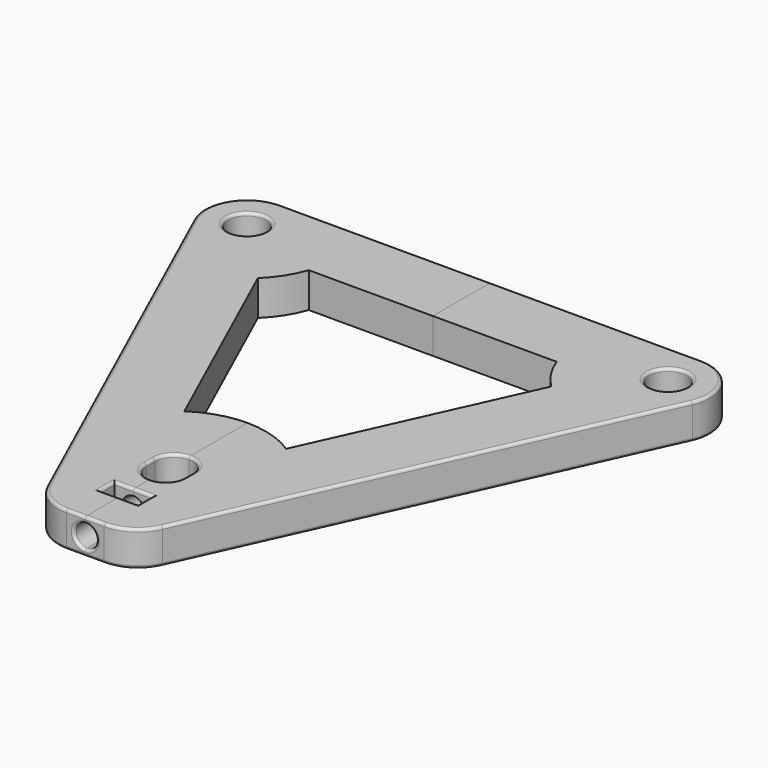
from build123d import *
from build123d import SkipClean  # not in build123d's __all__

# Parameters (mm, degrees)
F0_R          = 2.7
F1_DEPTH      = 5
F3_DEPTH      = 5
F5_END_RADIUS = 2.7
F4_R          = 1.6
F5_REACH      = 76.8264833996
F6_R          = 0.4


with BuildPart() as f1:
    # F0 (on Top) → F1 (new body)
    with BuildSketch(Plane.XY):
        with BuildLine():
            Line((0, -26.9), (0, 26.9))
            Line((0, 26.9), (-30, 26.9))
            ThreePointArc((-30, 26.9), (-35.0422077109, 24.1520979998), (-35.4659178703, 18.4253804667))
            Line((-35.4659178703, 18.4253804667), (-8.1659178703, -41.8746195333))
            ThreePointArc((-8.1659178703, -41.8746195333), (-5.9520979998, -44.4422077109), (-2.7, -45.4))
            Line((-2.7, -45.4), (0, -45.4))
            Line((0, -45.4), (0, -39.4))
            Line((0, -39.4), (-2.7, -39.4))
            Line((-2.7, -39.4), (-2.7, -36.8))
            Line((-2.7, -36.8), (0, -36.8))
            Line((0, -36.8), (0, -33.8))
            ThreePointArc((0, -33.8), (-1.9091883092, -33.0091883092), (-2.7, -31.1))
            Line((-2.7, -31.1), (-2.7, -29.6))
            ThreePointArc((-2.7, -29.6), (-1.9091883092, -27.6908116908), (0, -26.9))
        make_face()
        with Locations((-30, 20.9)):
            Circle(F0_R, mode=Mode.SUBTRACT)
    extrude(amount=F1_DEPTH)

    # F2 (on face) → F3 (cut, through all)
    with BuildSketch(Plane.XY.offset(5)):
        with BuildLine():
            Line((0, -16.5), (0, 16.5))
            Line((0, 16.5), (-17.6610373207, 16.5))
            ThreePointArc((-17.6610373207, 16.5), (-18.9911798312, 13.7995860339), (-20.9026205506, 11.4740948895))
            Line((-20.9026205506, 11.4740948895), (-7.2474182596, -18.687395885))
            ThreePointArc((-7.2474182596, -18.687395885), (-3.7851609011, -17.0587657325), (0, -16.5))
        make_face()
    extrude(amount=-F3_DEPTH, mode=Mode.SUBTRACT)

    f5_end = (Plane(origin=(0, -31.1, 2.5), x_dir=(-1, 0, 0), z_dir=(0, 0, -1)) * Cylinder(F5_END_RADIUS, 315.4959771518, mode=Mode.PRIVATE)).faces().sort_by_distance((-1.9091883092, -33.0091883092, 2.5))[0]
    # F4 (on face) → F5 (cut, up to the whole of a round face its end follows)
    with BuildSketch(Plane.XZ.offset(45.4)):
        with Locations((0, 2.5)):
            Circle(F4_R)
    f5_long = extrude(amount=-F5_REACH, mode=Mode.PRIVATE)
    add(split(f5_long, bisect_by=f5_end, keep=Keep.ALL, mode=Mode.PRIVATE).solids().sort_by_distance((0, -45.4, 2.5))[0], mode=Mode.SUBTRACT)

    # F6
    f6_edges = [f1.edges().sort_by_distance(p)[0] for p in [
        (-21.815918, -11.72462, 5),
        (-5.952098, -44.442208, 0),
        (-1.6, -45.4, 2.5),
        (-2.7, -38.1, 5),
        (-1.35, -39.4, 5),
        (-1.35, -36.8, 5),
        (-1.35, -39.4, 0),
        (-2.7, -38.1, 0),
        (-1.35, -36.8, 0),
        (-32.7, 20.9, 5),
        (-32.7, 20.9, 0),
        (-1.909188, -33.009188, 0),
        (-2.7, -30.35, 5),
    ]]
    fillet(f6_edges, radius=F6_R)

    # F7: F1 across face


with BuildPart() as f1_1:
    add(f1.part, clean=False)
    with SkipClean():  # cleaning this boolean's faces spoils the solid; the shape is the same uncleaned
        add(f1.part.mirror(Plane(origin=(0, 21.6932418104, 2.5), x_dir=(0, 1, 0), z_dir=(1, 0, 0))), clean=False)


solid = f1_1.part
